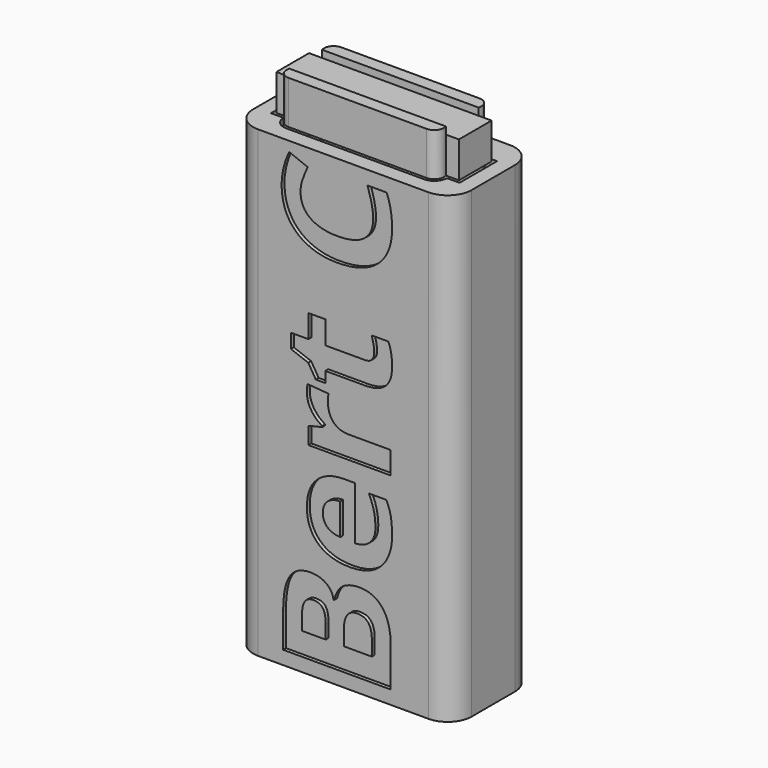
from build123d import *

# Parameters (mm, degrees)
F1_DEPTH     = 36.6
F0_W         = 0.7
F0_H         = 0.3
F0_W_2       = 0.25
F2_DEPTH     = 2
F3_TEXT_SIZE = 12.5426482535
F4_DEPTH     = 0.3
F6_DEPTH     = 3
F7_DEPTH     = 3.6


# Not quite as in the source:
# - a feature names something its author has since deleted; it is built from what else it names
# - Text() gives the source's letters only with a copy of the font that has no kerning and outlines rounded to 1/6400 em; it was checked with that copy


with BuildPart() as f1:
    # F0 (on Top) → F1 (new body)
    with BuildSketch(Plane.XY):
        with BuildLine():
            ThreePointArc((-9.1, -2.35), (-8.5142135624, -3.7642135624), (-7.1, -4.35))
            Line((-7.1, -4.35), (7.1, -4.35))
            ThreePointArc((7.1, -4.35), (8.5142135624, -3.7642135624), (9.1, -2.35))
            Line((9.1, -2.35), (9.1, 2.15))
            ThreePointArc((9.1, 2.15), (8.5142135624, 3.5642135624), (7.1, 4.15))
            Line((7.1, 4.15), (-7.1, 4.15))
            ThreePointArc((-7.1, 4.15), (-8.5142135624, 3.5642135624), (-9.1, 2.15))
            Line((-9.1, 2.15), (-9.1, -2.35))
        make_face()
        with BuildLine():
            Line((-7.85, 1.85), (-6.8, 1.85))
            ThreePointArc((-6.8, 1.85), (-6.4924621202, 2.5924621202), (-5.75, 2.9))
            Line((-5.75, 2.9), (5.75, 2.9))
            ThreePointArc((5.75, 2.9), (6.4924621202, 2.5924621202), (6.8, 1.85))
            Line((6.8, 1.85), (7.85, 1.85))
            Line((7.85, 1.85), (7.85, 0))
            Line((7.85, 0), (7.85, -2.05))
            Line((7.85, -2.05), (6.8, -2.05))
            ThreePointArc((6.8, -2.05), (6.4924621202, -2.7924621202), (5.75, -3.1))
            Line((5.75, -3.1), (-5.75, -3.1))
            ThreePointArc((-5.75, -3.1), (-6.4924621202, -2.7924621202), (-6.8, -2.05))
            Line((-6.8, -2.05), (-7.85, -2.05))
            Line((-7.85, -2.05), (-7.85, 0))
            Line((-7.85, 0), (-7.85, 1.85))
        make_face(mode=Mode.SUBTRACT)
    extrude(amount=F1_DEPTH)

    # F0 (on Top) → F2 (join)
    with BuildSketch(Plane.XY):
        with BuildLine():
            ThreePointArc((-9.1, -2.35), (-8.5142135624, -3.7642135624), (-7.1, -4.35))
            Line((-7.1, -4.35), (7.1, -4.35))
            ThreePointArc((7.1, -4.35), (8.5142135624, -3.7642135624), (9.1, -2.35))
            Line((9.1, -2.35), (9.1, 2.15))
            ThreePointArc((9.1, 2.15), (8.5142135624, 3.5642135624), (7.1, 4.15))
            Line((7.1, 4.15), (-7.1, 4.15))
            ThreePointArc((-7.1, 4.15), (-8.5142135624, 3.5642135624), (-9.1, 2.15))
            Line((-9.1, 2.15), (-9.1, -2.35))
        make_face()
        with BuildLine():
            Line((-7.85, 1.85), (-6.8, 1.85))
            ThreePointArc((-6.8, 1.85), (-6.4924621202, 2.5924621202), (-5.75, 2.9))
            Line((-5.75, 2.9), (5.75, 2.9))
            ThreePointArc((5.75, 2.9), (6.4924621202, 2.5924621202), (6.8, 1.85))
            Line((6.8, 1.85), (7.85, 1.85))
            Line((7.85, 1.85), (7.85, 0))
            Line((7.85, 0), (7.85, -2.05))
            Line((7.85, -2.05), (6.8, -2.05))
            ThreePointArc((6.8, -2.05), (6.4924621202, -2.7924621202), (5.75, -3.1))
            Line((5.75, -3.1), (-5.75, -3.1))
            ThreePointArc((-5.75, -3.1), (-6.4924621202, -2.7924621202), (-6.8, -2.05))
            Line((-6.8, -2.05), (-7.85, -2.05))
            Line((-7.85, -2.05), (-7.85, 0))
            Line((-7.85, 0), (-7.85, 1.85))
        make_face(mode=Mode.SUBTRACT)
        with BuildLine():
            Line((-6.1, -2.05), (-6.1, -0.4))
            Line((-6.1, -0.4), (-6.8, -0.4))
            Line((-6.8, -0.4), (-6.8, -1.2))
            Line((-6.8, -1.2), (-6.8, -2.05))
            ThreePointArc((-6.8, -2.05), (-6.4924621202, -2.7924621202), (-5.75, -3.1))
            Line((-5.75, -3.1), (5.75, -3.1))
            ThreePointArc((5.75, -3.1), (6.4924621202, -2.7924621202), (6.8, -2.05))
            Line((6.8, -2.05), (6.8, -1.2))
            Line((6.8, -1.2), (6.8, -0.4))
            Line((6.8, -0.4), (6.1, -0.4))
            Line((6.1, -0.4), (6.1, -2.05))
            ThreePointArc((6.1, -2.05), (5.9974873734, -2.2974873734), (5.75, -2.4))
            Line((5.75, -2.4), (-5.75, -2.4))
            ThreePointArc((-5.75, -2.4), (-5.9974873734, -2.2974873734), (-6.1, -2.05))
        make_face()
        with BuildLine():
            Line((-6.8, 0.2), (-6.1, 0.2))
            Line((-6.1, 0.2), (-6.1, 0.4))
            Line((-6.1, 0.4), (-6.1, 1.85))
            ThreePointArc((-6.1, 1.85), (-5.9974873734, 2.0974873734), (-5.75, 2.2))
            Line((-5.75, 2.2), (5.75, 2.2))
            ThreePointArc((5.75, 2.2), (5.9974873734, 2.0974873734), (6.1, 1.85))
            Line((6.1, 1.85), (6.1, 0.4))
            Line((6.1, 0.4), (6.1, 0.2))
            Line((6.1, 0.2), (6.8, 0.2))
            Line((6.8, 0.2), (6.8, 1))
            Line((6.8, 1), (6.8, 1.85))
            ThreePointArc((6.8, 1.85), (6.4924621202, 2.5924621202), (5.75, 2.9))
            Line((5.75, 2.9), (-5.75, 2.9))
            ThreePointArc((-5.75, 2.9), (-6.4924621202, 2.5924621202), (-6.8, 1.85))
            Line((-6.8, 1.85), (-6.8, 1))
            Line((-6.8, 1), (-6.8, 0.2))
        make_face()
        Polygon((-7.05, 0.2), (-6.8, 0.2), (-6.8, 1), (-6.8, 1.85), (-7.85, 1.85), (-7.85, 0), (-7.85, -2.05), (-6.8, -2.05), (-6.8, -1.2), (-6.8, -0.4), (-7.05, -0.4), (-7.05, -0.1), align=None)
        Polygon((6.8, 1), (6.8, 0.2), (7.05, 0.2), (7.05, -0.1), (7.05, -0.4), (6.8, -0.4), (6.8, -1.2), (6.8, -2.05), (7.85, -2.05), (7.85, 0), (7.85, 1.85), (6.8, 1.85), align=None)
        with Locations((-6.45, -0.25)):
            Rectangle(F0_W, F0_H)
        with Locations((-6.45, 0.05)):
            Rectangle(F0_W, F0_H)
        with Locations((6.45, 0.05)):
            Rectangle(F0_W, F0_H)
        with Locations((6.45, -0.25)):
            Rectangle(F0_W, F0_H)
        with Locations((-6.925, 0.05)):
            Rectangle(F0_W_2, F0_H)
        with Locations((-6.925, -0.25)):
            Rectangle(F0_W_2, F0_H)
        with Locations((6.925, 0.05)):
            Rectangle(F0_W_2, F0_H)
        with Locations((6.925, -0.25)):
            Rectangle(F0_W_2, F0_H)
    extrude(amount=-F2_DEPTH)

    # F3 (on face) → F4 (cut)
    with BuildSketch(Plane.XZ.offset(4.35)):
        with Locations(Location((3.9541067315, -2), (0, 0, 90))):
            Text('Bert C', F3_TEXT_SIZE, font='Open Sans', font_style=FontStyle.BOLD, text_align=(TextAlign.LEFT, TextAlign.BOTTOM))
    extrude(amount=-F4_DEPTH, mode=Mode.SUBTRACT)


with BuildPart() as f6:
    # F5 (on face) → F6 (new body)
    with BuildSketch(Plane.XY.offset(36.6)):
        with BuildLine():
            Line((6.5099342077, -1.8), (-6.5099342077, -1.8))
            ThreePointArc((-6.5099342077, -1.8), (-6.3980740698, -2.519041576), (-5.75, -2.85))
            Line((-5.75, -2.85), (5.75, -2.85))
            ThreePointArc((5.75, -2.85), (6.3980740698, -2.519041576), (6.5099342077, -1.8))
        make_face()
        Polygon((-7.6, -1.8), (-6.5099342077, -1.8), (6.5099342077, -1.8), (7.6, -1.8), (7.6, 1.6), (6.5099342077, 1.6), (-6.5099342077, 1.6), (-7.6, 1.6), align=None)
        with BuildLine():
            ThreePointArc((-5.75, 2.65), (-6.3980740698, 2.319041576), (-6.5099342077, 1.6))
            Line((-6.5099342077, 1.6), (6.5099342077, 1.6))
            ThreePointArc((6.5099342077, 1.6), (6.3980740698, 2.319041576), (5.75, 2.65))
            Line((5.75, 2.65), (-5.75, 2.65))
        make_face()
    extrude(amount=F6_DEPTH)

    # F5 (on face) → F7 (join)
    with BuildSketch(Plane.XY.offset(36.6)):
        with BuildLine():
            Line((6.5099342077, -1.8), (-6.5099342077, -1.8))
            ThreePointArc((-6.5099342077, -1.8), (-6.3980740698, -2.519041576), (-5.75, -2.85))
            Line((-5.75, -2.85), (5.75, -2.85))
            ThreePointArc((5.75, -2.85), (6.3980740698, -2.519041576), (6.5099342077, -1.8))
        make_face()
        with BuildLine():
            ThreePointArc((-5.75, 2.65), (-6.3980740698, 2.319041576), (-6.5099342077, 1.6))
            Line((-6.5099342077, 1.6), (6.5099342077, 1.6))
            ThreePointArc((6.5099342077, 1.6), (6.3980740698, 2.319041576), (5.75, 2.65))
            Line((5.75, 2.65), (-5.75, 2.65))
        make_face()
    extrude(amount=F7_DEPTH)


solid = Compound([f1.part, f6.part])
